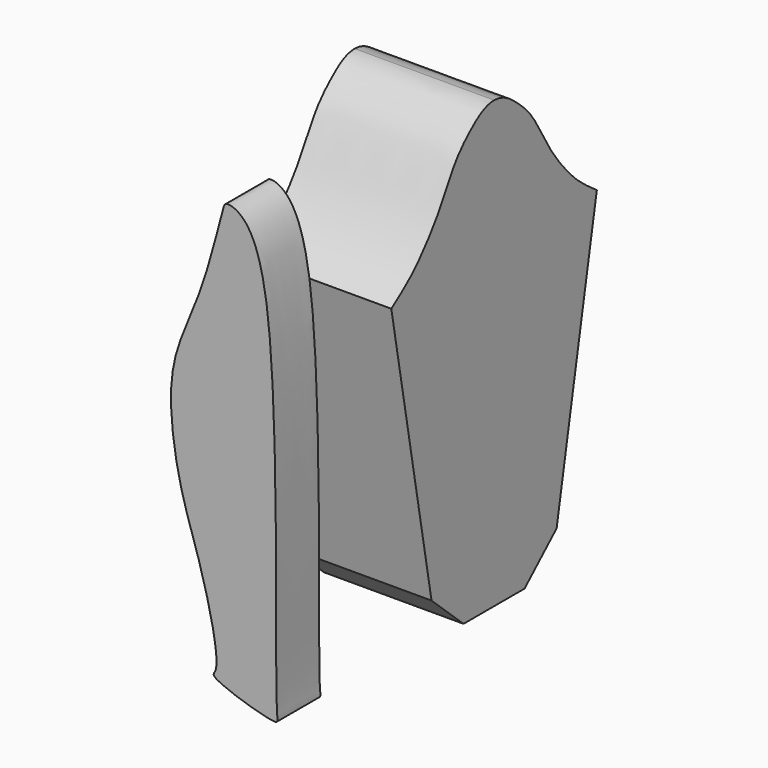
from build123d import *

# Parameters (mm, degrees)
F1_DEPTH  = 65
F5_R      = 3
F6_DEPTH  = 27
F8_SCALE  = 1.5
F11_DEPTH = 25
F12_SCALE = 1.5


# Not quite as in the source:
# - a feature of the source that left no trace in its solid (it failed there, or was rolled back) is left out


with BuildPart() as f1:
    # F0 (on Right) → F1 (new body)
    with BuildSketch(Plane.YZ):
        with BuildLine():
            add(Edge.make_bspline(
                [(0, 116.170451045), (0.9828145316, 116.098523156), (3.2124722619, 115.9353442766), (8.0579268571, 114.0720893794), (14.6187789397, 108.775157515), (23.1603373895, 100.5582162883), (31.6909696821, 83.1334415189), (42.0097439258, 70.0417832015), (49.7783168483, 62.0961919241), (56.4237470409, 57.3854542674), (59.8379671574, 54.9652203918)],
                knots=[0, 0, 0, 0, 0.0686098354, 0.155651392, 0.2675662145, 0.4017654935, 0.5745697868, 0.7344591888, 0.8635731995, 1, 1, 1, 1], degree=3))
            add(Edge.make_bspline(
                [(0, 116.170451045), (-0.9828145316, 116.098523156), (-3.2124722619, 115.9353442766), (-8.0579268571, 114.0720893794), (-14.6187789397, 108.775157515), (-23.1603373895, 100.5582162883), (-31.6909696821, 83.1334415189), (-42.0097439258, 70.0417832015), (-49.7783168483, 62.0961919241), (-56.4237470409, 57.3854542674), (-59.8379671574, 54.9652203918)],
                knots=[0, 0, 0, 0, 0.0686098354, 0.155651392, 0.2675662145, 0.4017654935, 0.5745697868, 0.7344591888, 0.8635731995, 1, 1, 1, 1], degree=3))
            Line((-59.8379671574, 54.9652203918), (-36.4224053919, -74.2475837469))
            Line((-36.4224053919, -74.2475837469), (-17.776966095, -91.3761481643))
            Line((-17.776966095, -91.3761481643), (0, -91.3761481643))
            Line((0, -91.3761481643), (17.776966095, -91.3761481643))
            Line((17.776966095, -91.3761481643), (36.4224053919, -74.2475837469))
            Line((36.4224053919, -74.2475837469), (59.8379671574, 54.9652203918))
        make_face()
    extrude(amount=F1_DEPTH)


with BuildPart() as f6:
    # F5 (on offset) → F6 (new body)
    with BuildSketch(Plane.XY.offset(-78)):
        with Locations((36.8607869876, 0)):
            Circle(F5_R)
    extrude(amount=-F6_DEPTH)


with BuildPart() as f1_1:
    # F8: moved
    add(f1.part.scale(F8_SCALE))


with BuildPart() as f11:
    # F10 (on offset) → F11 (new body)
    with BuildSketch(Plane.XZ.offset(104)):
        with BuildLine():
            add(Edge.make_bspline(
                [(43.4212864901, 119.0287297239), (44.5590829036, 119.445319306), (51.895794014, 117.7035317815), (70.0536524909, 88.2179731004), (65.2706911825, -79.6441995386), (68.5031285729, -88.2168032625), (33.9713508157, -77.2553782815), (41.5970331679, -73.2863722888), (31.3204411062, -30.0524753033), (21.3458190874, -5.732934009), (13.8975667347, 44.070003515), (31.7630651573, 75.0287070352), (41.2673378658, 114.5874505068), (42.4764196168, 118.6827788217), (43.4212864901, 119.0287297239)],
                knots=[0, 0, 0, 0, 0.0368658424, 0.1293943223, 0.3339880245, 0.3643937432, 0.4501249655, 0.4778219637, 0.5776561287, 0.6665716107, 0.7729255556, 0.8714697753, 0.9693852848, 1, 1, 1, 1], degree=3))
        make_face()
    extrude(amount=F11_DEPTH)


with BuildPart() as f11_1:
    # F12: moved
    add(f11.part.scale(F12_SCALE))


solid = Compound([f1_1.part, f11_1.part])
